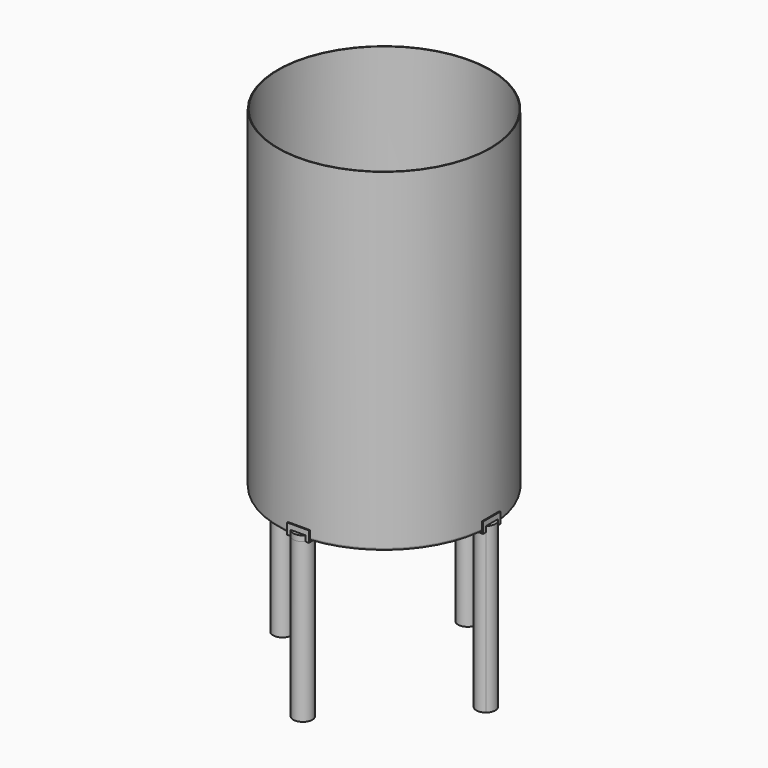
from build123d import *
from build123d import SkipClean  # not in build123d's __all__

# Parameters (mm, degrees)
F0_R           = 490
F1_DEPTH       = 1535
F2_T           = -3
F3_R           = 10
F5_W           = 100
F5_H           = 50
F6_DEPTH       = 5
F7_W           = 100
F7_H           = 5
F8_DEPTH       = 50
F10_W          = 100
F10_H          = 50
F11_DEPTH      = 5
F12_W          = 100
F12_H          = 5
F13_DEPTH      = 50
F15_W          = 100
F15_H          = 50
F16_DEPTH      = 5
F17_W          = 100
F17_H          = 5
F18_DEPTH      = 50
F20_W          = 100
F20_H          = 50
F21_DEPTH      = 5
F22_W          = 100
F22_H          = 5
F23_DEPTH      = 25.4
F25_DEPTH      = 730
F25_DEPTH_BACK = 25.4
F24_R          = 43.75
F26_DEPTH      = 730
F27_R          = 43.75
F28_DEPTH      = 730
F30_DEPTH      = 25.4
F31_R          = 43.75
F32_DEPTH      = 730
F34_DEPTH      = 25.4
F35_R          = 43.75
F36_DEPTH      = 730
F38_DEPTH      = 25.4
F39_R          = 25
F40_DEPTH      = 25.4


with BuildPart() as f1:
    # F0 (on Top) → F1 (new body)
    with BuildSketch(Plane.XY):
        Circle(F0_R)
    extrude(amount=F1_DEPTH)

    # F2
    f2_openings = [f1.faces().sort_by_distance(p)[0] for p in [
        (0, 0, 1535),
    ]]
    offset(amount=F2_T, openings=f2_openings)

    # F3
    f3_edges = [f1.edges().sort_by_distance(p)[0] for p in [
        (-490, 0, 0),
    ]]
    fillet(f3_edges, radius=F3_R)

    # F39 (on face) → F40 (cut)
    with BuildSketch(Plane.XY.offset(3)):
        Circle(F39_R)
    extrude(amount=-F40_DEPTH, mode=Mode.SUBTRACT)


with BuildPart() as f6:
    # F5 (on offset) → F6 (new body)
    with BuildSketch(Plane.XZ.offset(490.0168)):
        with Locations((0, 20)):
            Rectangle(F5_W, F5_H)
    extrude(amount=F6_DEPTH)

    # F7 (on face) → F8 (join)
    with BuildSketch(Plane(origin=(0, -490.0168, 0), x_dir=(-1, 0, 0), z_dir=(0, 1, 0))):
        with Locations((0, -2.5)):
            Rectangle(F7_W, F7_H)
    extrude(amount=F8_DEPTH)

    # F27 (on face) → F28 (join)
    with BuildSketch(Plane(origin=(0, 0, -5), x_dir=(1, 0, 0), z_dir=(0, 0, -1))):
        with Locations((0, 467.5168)):
            Circle(F27_R)
    extrude(amount=F28_DEPTH)

    # F29 (on face) → F30 (join)
    with BuildSketch(Plane.XY.offset(-5)):
        with BuildLine():
            Line((34.026643972, -495.0168), (-34.026643972, -495.0168))
            ThreePointArc((-34.026643972, -495.0168), (0, -511.2668), (34.026643972, -495.0168))
        make_face()
    extrude(amount=F30_DEPTH)


with BuildPart() as f11:
    # F10 (on offset) → F11 (new body)
    with BuildSketch(Plane.YZ.offset(490.474)):
        with Locations((0, 20)):
            Rectangle(F10_W, F10_H)
    extrude(amount=F11_DEPTH)

    # F12 (on face) → F13 (join)
    with BuildSketch(Plane(origin=(490.474, 0, 0), x_dir=(0, -1, 0), z_dir=(-1, 0, 0))):
        with Locations((0, -2.5)):
            Rectangle(F12_W, F12_H)
    extrude(amount=F13_DEPTH)

    # F24 (on face) → F25 (join, two sides)
    with BuildSketch(Plane(origin=(0, 0, -5), x_dir=(1, 0, 0), z_dir=(0, 0, -1))) as f25_sk:
        with BuildLine():
            ThreePointArc((495.474, -34.026643972), (507.4530292434, -18.8538789112), (511.724, 0))
            ThreePointArc((511.724, 0), (507.4530292434, 18.8538789112), (495.474, 34.026643972))
            Line((495.474, 34.026643972), (495.474, -34.026643972))
        make_face()
    extrude(amount=F25_DEPTH)
    extrude(f25_sk.sketch, amount=-F25_DEPTH_BACK)

    # F24 (on face) → F26 (join)
    with BuildSketch(Plane(origin=(0, 0, -5), x_dir=(1, 0, 0), z_dir=(0, 0, -1))):
        with Locations((467.974, 0)):
            Circle(F24_R)
    extrude(amount=F26_DEPTH)


with BuildPart() as f16:
    # F15 (on offset) → F16 (new body)
    with BuildSketch(Plane.YZ.offset(-490.0168)):
        with Locations((0, 20)):
            Rectangle(F15_W, F15_H)
    extrude(amount=-F16_DEPTH)

    # F17 (on face) → F18 (join)
    with BuildSketch(Plane.YZ.offset(-490.0168)):
        with Locations((0, -2.5)):
            Rectangle(F17_W, F17_H)
    extrude(amount=F18_DEPTH)

    # F31 (on face) → F32 (join)
    with BuildSketch(Plane(origin=(0, 0, -5), x_dir=(1, 0, 0), z_dir=(0, 0, -1))):
        with Locations((-467.5168, 0)):
            Circle(F31_R)
    extrude(amount=F32_DEPTH)

    # F33 (on face) → F34 (join)
    with BuildSketch(Plane.XY.offset(-5)):
        with BuildLine():
            Line((-495.0168, -34.026643972), (-495.0168, 34.026643972))
            ThreePointArc((-495.0168, 34.026643972), (-511.2668, 0), (-495.0168, -34.026643972))
        make_face()
    with SkipClean():  # cleaning this boolean's faces spoils the solid; the shape is the same uncleaned
        extrude(amount=F34_DEPTH)


with BuildPart() as f21:
    # F20 (on offset) → F21 (new body)
    with BuildSketch(Plane.XZ.offset(-490.0676)):
        with Locations((0, 20)):
            Rectangle(F20_W, F20_H)
    extrude(amount=-F21_DEPTH)

    # F22 (on face) → F23 (join)
    with BuildSketch(Plane.XZ.offset(-490.0676)):
        with Locations((0, -2.5)):
            Rectangle(F22_W, F22_H)
    extrude(amount=F23_DEPTH)

    # F35 (on face) → F36 (join)
    with BuildSketch(Plane(origin=(0, 0, -5), x_dir=(1, 0, 0), z_dir=(0, 0, -1))):
        with Locations((0, -479.8676)):
            Circle(F35_R)
    extrude(amount=F36_DEPTH)

    # F37 (on face) → F38 (join)
    with BuildSketch(Plane.XY.offset(-5)):
        with BuildLine():
            Line((-41.0246572198, 495.0676), (41.0246572198, 495.0676))
            ThreePointArc((41.0246572198, 495.0676), (0, 523.6176), (-41.0246572198, 495.0676))
        make_face()
    extrude(amount=F38_DEPTH)


solid = Compound([f1.part, f6.part, f11.part, f16.part, f21.part])
